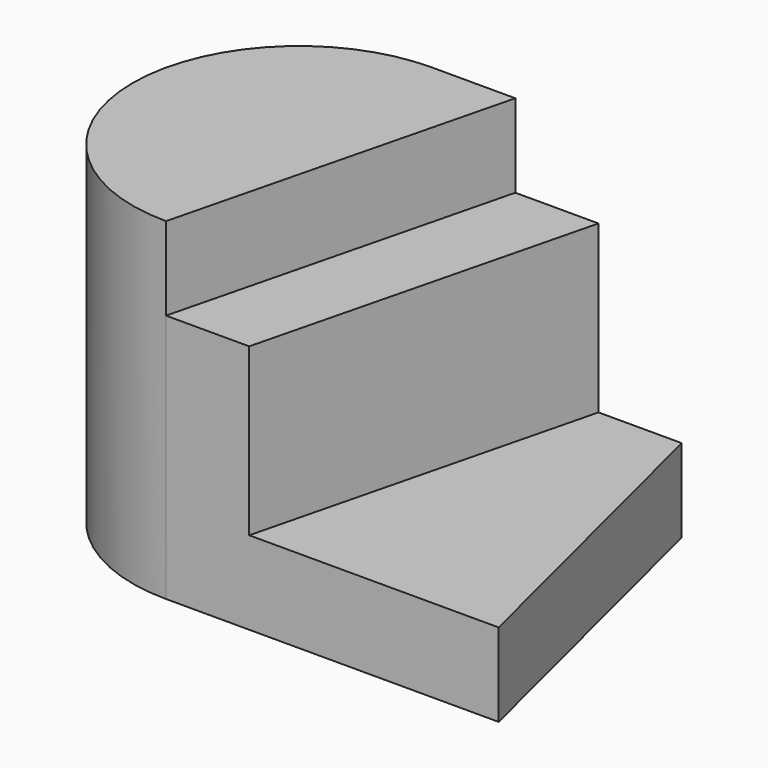
from build123d import *

# Parameters (mm, degrees)
F0_W     = 60
F0_H     = 40
F1_DEPTH = 40
F2_R     = 19.99999
F4_DEPTH = 40
F6_DEPTH = 30
F8_DEPTH = 10


# Not quite as in the source:
# - a fillet or chamfer is up to 0.001 mm smaller than in the source, because OpenCascade refuses the exact size


with BuildPart() as f1:
    # F0 (on Top) → F1 (new body)
    with BuildSketch(Plane.XY):
        with Locations((30, 20)):
            Rectangle(F0_W, F0_H)
    extrude(amount=F1_DEPTH)

    # F2 (radius 20 in the source; OpenCascade refuses exactly that, so slightly less here)
    f2_edges = [f1.edges().sort_by_distance(p)[0] for p in [
        (0, 40, 20),
        (0, 0, 20),
    ]]
    fillet(f2_edges, radius=F2_R)

    # F3 (on face) → F4 (cut)
    with BuildSketch(Plane.XY.offset(40)):
        Polygon((60, 0), (60, 40), (50, 40), align=None)
    extrude(amount=-F4_DEPTH, mode=Mode.SUBTRACT)

    # F5 (on face) → F6 (cut)
    with BuildSketch(Plane.XY.offset(40)):
        Polygon((60, 0), (50, 40), (40, 40), (30, 0), align=None)
    extrude(amount=-F6_DEPTH, mode=Mode.SUBTRACT)

    # F7 (on face) → F8 (cut)
    with BuildSketch(Plane.XY.offset(40)):
        Polygon((30, 0), (40, 40), (30, 40), (20, 0), align=None)
    extrude(amount=-F8_DEPTH, mode=Mode.SUBTRACT)


solid = f1.part
